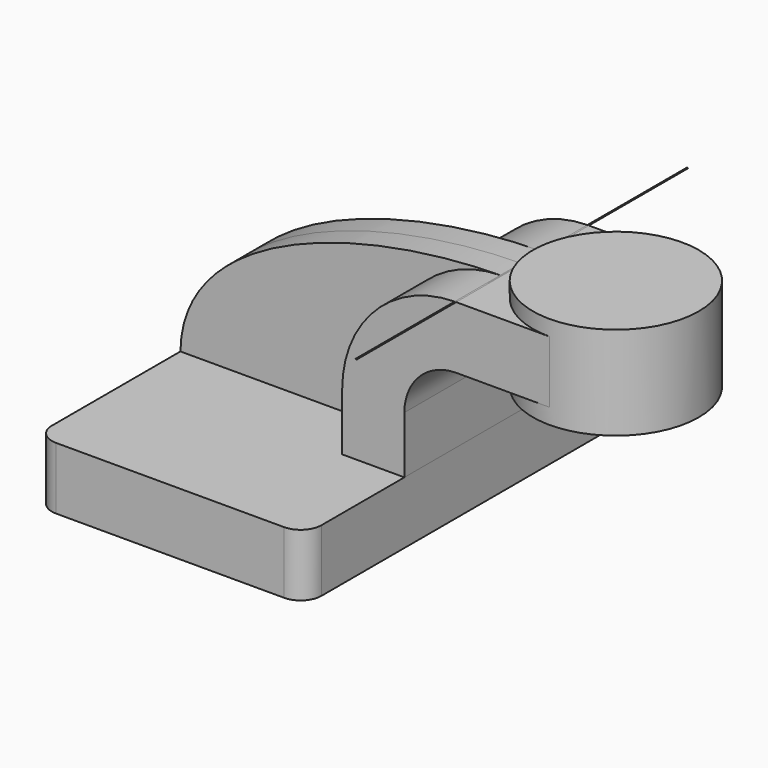
from build123d import *

# Parameters (mm, degrees)
F1_DEPTH = 63.5
F0_W     = 25.4
F0_H     = 19.05
F2_DEPTH = 25.4
F3_DEPTH = 7.9375
F5_R     = 6.35


with BuildPart() as f1:
    # F0 (on Front) → F1 (new body, symmetric)
    with BuildSketch(Plane.XZ):
        Polygon((-41.275, -9.525), (41.275, -9.525), (41.275, 9.525), (22.225, 9.525), (-41.275, 9.525), align=None)
    extrude(amount=F1_DEPTH, both=True)

    # F5
    f5_edges = [f1.edges().sort_by_distance(p)[0] for p in [
        (41.275, -63.5, 0),
        (-41.275, -63.5, 0),
        (41.275, 63.5, 0),
        (-41.275, 63.5, 0),
    ]]
    fillet(f5_edges, radius=F5_R)


with BuildPart() as f1b:
    # F0 (on Front) → F1, piece 2 (new body, symmetric)
    with BuildSketch(Plane.XZ):
        with BuildLine():
            ThreePointArc((57.15, 61.9252), (56.9143112761, 61.9244047272), (56.6786332859, 61.9220189449))
            add(Edge.make_bspline(
                [(56.6786332859, 61.9220189449), (56.8358800851, 61.9232946855), (56.9930032828, 61.9243550243), (57.15, 61.9252)],
                knots=[111.1070273271, 111.1070273271, 111.1070273271, 111.1070273271, 111.5045361635, 111.5045361635, 111.5045361635, 111.5045361635], degree=3))
        make_face()
    extrude(amount=F1_DEPTH, both=True)


with BuildPart() as f2:
    # F0 (on Front) → F2 (new body, symmetric)
    with BuildSketch(Plane.XZ):
        with BuildLine():
            Line((22.225, 9.525), (41.275, 9.525))
            Line((41.275, 9.525), (41.275, 27.0002))
            ThreePointArc((41.275, 27.0002), (45.9246798487, 38.2255201513), (57.15, 42.8752))
            Line((57.15, 42.8752), (60.325, 42.8752))
            Line((60.325, 42.8752), (60.325, 61.9252))
            Line((60.325, 61.9252), (57.15, 61.9252))
            add(Edge.make_bspline(
                [(56.6786332859, 61.9220189449), (56.8358800851, 61.9232946855), (56.9930032828, 61.9243550243), (57.15, 61.9252)],
                knots=[111.1070273271, 111.1070273271, 111.1070273271, 111.1070273271, 111.5045361635, 111.5045361635, 111.5045361635, 111.5045361635], degree=3))
            ThreePointArc((56.6786332859, 61.9220189449), (32.288200915, 51.5286848952), (22.225, 27.0002))
            Line((22.225, 27.0002), (22.225, 9.525))
        make_face()
        with Locations((73.025, 52.4002)):
            Rectangle(F0_W, F0_H)
    extrude(amount=F2_DEPTH, both=True)

    # F0 (on Front) → F4 (revolve)
    with BuildSketch(Plane.XZ):
        Polygon((85.725, 61.9252), (85.725, 42.8752), (85.725, 38.1), (111.125, 38.1), (111.125, 66.675), (85.725, 66.675), align=None)
    revolve(axis=Axis((85.725, 0, 52.3875), (0, 0, -1)))


with BuildPart() as f3:
    # F0 (on Front) → F3 (new body, symmetric)
    with BuildSketch(Plane.XZ):
        with BuildLine():
            add(Edge.make_bspline(
                [(-41.275, 9.525), (-40.8812896935, 44.3806199312), (12.726844531, 61.565438842), (56.6786332859, 61.9220189449)],
                knots=[0, 0, 0, 0, 111.1070273271, 111.1070273271, 111.1070273271, 111.1070273271], degree=3))
            Line((-41.275, 9.525), (22.225, 9.525))
            Line((22.225, 9.525), (22.225, 27.0002))
            ThreePointArc((22.225, 27.0002), (32.288200915, 51.5286848952), (56.6786332859, 61.9220189449))
        make_face()
    extrude(amount=F3_DEPTH, both=True)


solid = Compound([f1.part, f1b.part, f2.part, f3.part])
